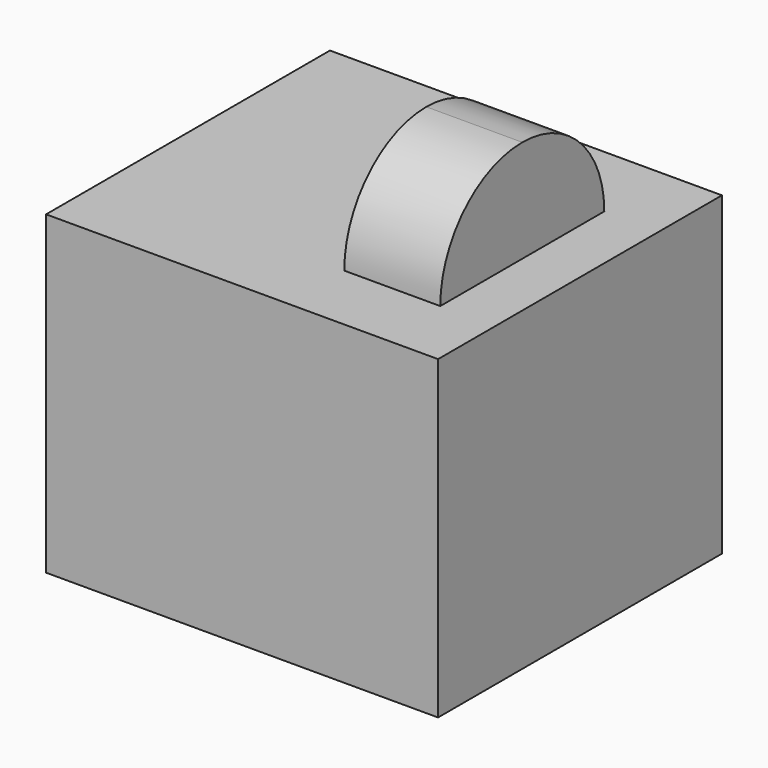
from build123d import *

# Parameters (mm, degrees)
F0_W     = 103.7199497223
F0_H     = 93.8791483641
F1_DEPTH = 83.4754128009
F5_DEPTH = 25.4


with BuildPart() as f1:
    # F0 (on Top) → F1 (new body)
    with BuildSketch(Plane.XY):
        with Locations((4.3902695179, -5.4262652993)):
            Rectangle(F0_W, F0_H)
    extrude(amount=F1_DEPTH)

    # F4 (on face) → F5 (join)
    with BuildSketch(Plane(origin=(41.7745485902, 0, 0), x_dir=(0, -1, 0), z_dir=(-1, 0, 0))):
        with BuildLine():
            ThreePointArc((33.5486456752, 83.4754128009), (25.6043620093, 102.6546101703), (6.4251646399, 110.5988938361))
            Line((6.4251646399, 110.5988938361), (6.4251646399, 83.4754128009))
            Line((6.4251646399, 83.4754128009), (33.5486456752, 83.4754128009))
        make_face()
        with BuildLine():
            Line((6.4251646399, 83.4754128009), (6.4251646399, 110.5988938361))
            ThreePointArc((6.4251646399, 110.5988938361), (-12.7540327294, 102.6546101703), (-20.6983163953, 83.4754128009))
            Line((-20.6983163953, 83.4754128009), (6.4251646399, 83.4754128009))
        make_face()
    extrude(amount=F5_DEPTH)


solid = f1.part
